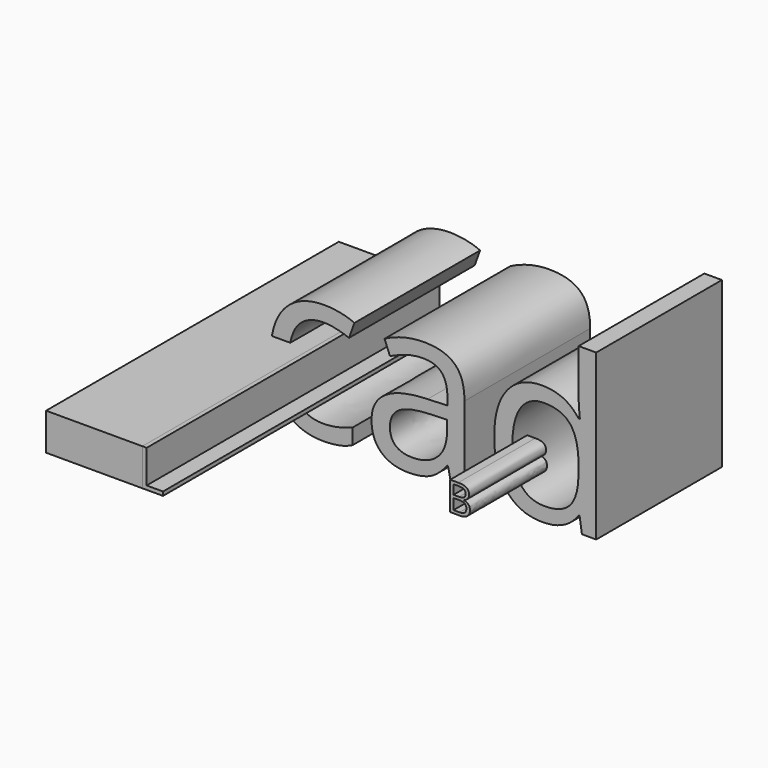
from build123d import *

# Parameters (mm, degrees)
F0_TEXT_SIZE = 56.257013542
F1_DEPTH     = 40.8
F2_TEXT_SIZE = 13.4682489766
F3_DEPTH     = 25
F4_TEXT_SIZE = 6.9594722138
F5_DEPTH     = 25
F6_TEXT_SIZE = 10.374483342
F7_DEPTH     = 25
F8_DEPTH     = 30
F9_DEPTH     = 20
F10_DEPTH    = 20
F11_DEPTH    = 25


# Not quite as in the source:
# - Text() gives the source's letters only with a copy of the font that has no kerning and outlines rounded to 1/6400 em; it was checked with that copy


with BuildPart() as f1:
    # F0 (on Front) → F1 (new body)
    with BuildSketch(Plane.XZ):
        with Locations((-32.1843548684, 0)):
            Text('cad', F0_TEXT_SIZE, font='Open Sans', text_align=(TextAlign.LEFT, TextAlign.BOTTOM))
    extrude(amount=F1_DEPTH)


with BuildPart() as f3:
    # F2 (on Front) → F3 (new body)
    with BuildSketch(Plane.XZ):
        with Locations((-20.2901829034, 9.5215793699)):
            Text('L', F2_TEXT_SIZE, font='Open Sans', text_align=(TextAlign.LEFT, TextAlign.BOTTOM))
    extrude(amount=F3_DEPTH)

    # F8 (add): a face of the model
    f8_faces = [f3.faces().sort_by_distance(p)[0] for p in [
        (-18.8585298678, -25, 14.3291129304),
    ]]
    extrude(f8_faces, amount=F8_DEPTH)

    # F9 (add): a face of the model
    f9_faces = [f3.faces().sort_by_distance(p)[0] for p in [
        (-18.8585298678, -55, 14.3291129304),
    ]]
    extrude(f9_faces, amount=F9_DEPTH)

    # F10 (add): a face of the model
    f10_faces = [f3.faces().sort_by_distance(p)[0] for p in [
        (-18.8585298678, -75, 14.3291129304),
    ]]
    extrude(f10_faces, amount=F10_DEPTH)


with BuildPart() as f5:
    # F4 (on Front) → F5 (new body)
    with BuildSketch(Plane.XZ):
        with Locations((7.5051845051, 6.3307303935)):
            Text('A', F4_TEXT_SIZE, font='Open Sans', text_align=(TextAlign.LEFT, TextAlign.BOTTOM))
    extrude(amount=F5_DEPTH)


with BuildPart() as f7:
    # F6 (on face) → F7 (new body)
    with BuildSketch(Plane.XZ.offset(40.8)):
        with Locations((36.5853868425, 10.6098745018)):
            Text('B', F6_TEXT_SIZE, font='Open Sans', text_align=(TextAlign.LEFT, TextAlign.BOTTOM))
    extrude(amount=F7_DEPTH)


with BuildPart() as f11:
    # F11 (new): a face of the model
    f11_faces = [f3.part.faces().sort_by_distance(p)[0] for p in [
        (-18.9686109726, -47.5, 14.3291129304),
    ]]
    extrude(f11_faces, amount=F11_DEPTH)


solid = Compound([f1.part, f3.part, f5.part, f7.part, f11.part])
